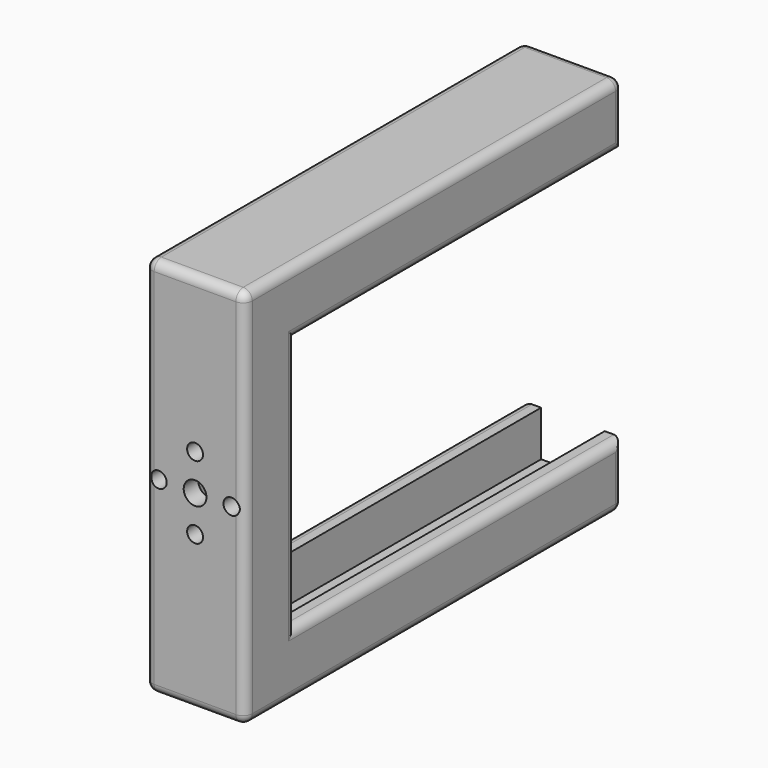
from build123d import *

# Parameters (mm, degrees)
F0_W          = 22
F0_H          = 84
F0_W_2        = 14
F0_H_2        = 76
F1_DEPTH      = 100
F2_W          = 22
F2_H          = 84
F3_DEPTH      = 4
F4_R          = 2.5
F4_R_2        = 1.75
F5_DEPTH      = 13
F6_W          = 90
F6_H          = 56
F7_DEPTH      = 22.001
F8_T1_DEPTH   = 100
F8_T3_DEPTH   = 17
F8_T5_DEPTH   = 95
F8_T7_DEPTH   = 56
F8_T9_DEPTH   = 17
F8_T11_DEPTH  = 80
F8_T13_DEPTH  = 18
F8_S17_W      = 2
F8_S17_H      = 2
F8_T18_DEPTH  = 2
F8_S23_W      = 2
F8_S23_H      = 2
F8_T24_DEPTH  = 2
F8_S29_W      = 2
F8_S29_H      = 2
F8_T30_DEPTH  = 2
F8_S35_W      = 2
F8_S35_H      = 2
F8_T36_DEPTH  = 2
F8_S41_W      = 2
F8_S41_H      = 2
F8_T42_DEPTH  = 2
F8_S47_W      = 2
F8_S47_H      = 2
F8_T48_DEPTH  = 2
F8_S53_W      = 2
F8_S53_H      = 2
F8_T54_DEPTH  = 2
F8_S59_W      = 2
F8_S59_H      = 2
F8_T60_DEPTH  = 2
F8_T67_DEPTH  = 100
F8_T71_DEPTH  = 61
F8_T78_DEPTH  = 61
F8_T82_DEPTH  = 100
F8_T89_DEPTH  = 100
F8_T93_DEPTH  = 61
F8_T100_DEPTH = 61
F8_T104_DEPTH = 100


# Not quite as in the source:
# - a fillet or chamfer that OpenCascade refuses, or shapes differently, is made with other operations: its cross-section is extruded or revolved along the edge and cut away or added


with BuildPart() as f1:
    # F0 (on Front) → F1 (new body)
    with BuildSketch(Plane.XZ):
        Rectangle(F0_W, F0_H)
        Rectangle(F0_W_2, F0_H_2, mode=Mode.SUBTRACT)
    extrude(amount=F1_DEPTH)

    # F2 (on face) → F3 (join)
    with BuildSketch(Plane.XZ.offset(100)):
        Rectangle(F2_W, F2_H)
    extrude(amount=F3_DEPTH)

    # F4 (on face) → F5 (cut)
    with BuildSketch(Plane.XZ.offset(104)):
        Circle(F4_R)
        with Locations((0, 8)):
            Circle(F4_R_2)
        with Locations((-8, 0)):
            Circle(F4_R_2)
        with Locations((0, -8)):
            Circle(F4_R_2)
        with Locations((8, 0)):
            Circle(F4_R_2)
    extrude(amount=-F5_DEPTH, mode=Mode.SUBTRACT)

    # F6 (on face) → F7 (cut, through all)
    with BuildSketch(Plane.YZ.offset(11)):
        with Locations((-45, 0)):
            Rectangle(F6_W, F6_H)
    extrude(amount=-F7_DEPTH, mode=Mode.SUBTRACT)

    # F8: fillet of radius 2 on 20 edges, made by hand

    # F8_s2 → F8_t1 (cut)
    with BuildSketch(Plane.XZ.offset(2)):
        with BuildLine():
            ThreePointArc((11, -40), (10.4142135624, -41.4142135624), (9, -42))
            Line((9, -42), (11, -42))
            Line((11, -42), (11, -40))
        make_face()
        with BuildLine():
            ThreePointArc((9, 42), (10.4142135624, 41.4142135624), (11, 40))
            Line((11, 40), (11, 42))
            Line((11, 42), (9, 42))
        make_face()
        with BuildLine():
            ThreePointArc((-11, -40), (-10.4142135624, -41.4142135624), (-9, -42))
            Line((-9, -42), (-11, -42))
            Line((-11, -42), (-11, -40))
        make_face()
        with BuildLine():
            ThreePointArc((-9, 42), (-10.4142135624, 41.4142135624), (-11, 40))
            Line((-11, 40), (-11, 42))
            Line((-11, 42), (-9, 42))
        make_face()
    extrude(amount=F8_T1_DEPTH, mode=Mode.SUBTRACT)

    # F8_s4 → F8_t3 (cut)
    with BuildSketch(Plane.XY.offset(-40)):
        with BuildLine():
            ThreePointArc((11, -2), (10.4142135624, -0.5857864376), (9, 0))
            Line((9, 0), (11, 0))
            Line((11, 0), (11, -2))
        make_face()
        with BuildLine():
            ThreePointArc((-11, -2), (-10.4142135624, -0.5857864376), (-9, 0))
            Line((-9, 0), (-11, 0))
            Line((-11, 0), (-11, -2))
        make_face()
    extrude(amount=F8_T3_DEPTH, mode=Mode.SUBTRACT)

    # F8_s6 → F8_t5 (cut)
    with BuildSketch(Plane.XZ.offset(-5)):
        with BuildLine():
            ThreePointArc((11, -30), (10.4142135624, -28.5857864376), (9, -28))
            Line((9, -28), (11, -28))
            Line((11, -28), (11, -30))
        make_face()
        with BuildLine():
            ThreePointArc((11, 30), (10.4142135624, 28.5857864376), (9, 28))
            Line((9, 28), (11, 28))
            Line((11, 28), (11, 30))
        make_face()
        with BuildLine():
            ThreePointArc((-11, 30), (-10.4142135624, 28.5857864376), (-9, 28))
            Line((-9, 28), (-11, 28))
            Line((-11, 28), (-11, 30))
        make_face()
        with BuildLine():
            ThreePointArc((-11, -30), (-10.4142135624, -28.5857864376), (-9, -28))
            Line((-9, -28), (-11, -28))
            Line((-11, -28), (-11, -30))
        make_face()
    extrude(amount=F8_T5_DEPTH, mode=Mode.SUBTRACT)

    # F8_s8 → F8_t7 (cut)
    with BuildSketch(Plane.XY.offset(-28)):
        with BuildLine():
            ThreePointArc((11, -92), (10.4142135624, -90.5857864376), (9, -90))
            Line((9, -90), (11, -90))
            Line((11, -90), (11, -92))
        make_face()
        with BuildLine():
            ThreePointArc((-11, -92), (-10.4142135624, -90.5857864376), (-9, -90))
            Line((-9, -90), (-11, -90))
            Line((-11, -90), (-11, -92))
        make_face()
    extrude(amount=F8_T7_DEPTH, mode=Mode.SUBTRACT)

    # F8_s10 → F8_t9 (cut)
    with BuildSketch(Plane.XY.offset(23)):
        with BuildLine():
            ThreePointArc((11, -2), (10.4142135624, -0.5857864376), (9, 0))
            Line((9, 0), (11, 0))
            Line((11, 0), (11, -2))
        make_face()
        with BuildLine():
            ThreePointArc((-11, -2), (-10.4142135624, -0.5857864376), (-9, 0))
            Line((-9, 0), (-11, 0))
            Line((-11, 0), (-11, -2))
        make_face()
    extrude(amount=F8_T9_DEPTH, mode=Mode.SUBTRACT)

    # F8_s12 → F8_t11 (cut)
    with BuildSketch(Plane.XY.offset(-40)):
        with BuildLine():
            ThreePointArc((11, -102), (10.4142135624, -103.4142135624), (9, -104))
            Line((9, -104), (11, -104))
            Line((11, -104), (11, -102))
        make_face()
        with BuildLine():
            ThreePointArc((-9, -104), (-10.4142135624, -103.4142135624), (-11, -102))
            Line((-11, -102), (-11, -104))
            Line((-11, -104), (-9, -104))
        make_face()
    extrude(amount=F8_T11_DEPTH, mode=Mode.SUBTRACT)

    # F8_s14 → F8_t13 (cut)
    with BuildSketch(Plane.YZ.offset(-9)):
        with BuildLine():
            ThreePointArc((-102, 42), (-103.4142135624, 41.4142135624), (-104, 40))
            Line((-104, 40), (-104, 42))
            Line((-104, 42), (-102, 42))
        make_face()
        with BuildLine():
            ThreePointArc((-2, 42), (-0.5857864376, 41.4142135624), (0, 40))
            Line((0, 40), (0, 42))
            Line((0, 42), (-2, 42))
        make_face()
        with BuildLine():
            ThreePointArc((-104, -40), (-103.4142135624, -41.4142135624), (-102, -42))
            Line((-102, -42), (-104, -42))
            Line((-104, -42), (-104, -40))
        make_face()
        with BuildLine():
            ThreePointArc((-2, -42), (-0.5857864376, -41.4142135624), (0, -40))
            Line((0, -40), (0, -42))
            Line((0, -42), (-2, -42))
        make_face()
    extrude(amount=F8_T13_DEPTH, mode=Mode.SUBTRACT)


with BuildPart() as f8_tool16:
    # F8_s17 → F8_t18 (new body)
    with BuildSketch(Plane.YZ.offset(9)):
        with Locations((-103, -41)):
            Rectangle(F8_S17_W, F8_S17_H)
    extrude(amount=F8_T18_DEPTH)

    # F8_s19 → F8_t20 (revolve, cut)
    with BuildSketch(Plane(origin=(9, -102, -40), x_dir=(0, 0.7071067812, 0.7071067812), z_dir=(0, 0.7071067812, -0.7071067812))):
        with BuildLine():
            ThreePointArc((0, -2), (2, 0), (0, 2))
            Line((0, 2), (0, -2))
        make_face()
    revolve(axis=Axis((9, -102, -40), (1, 0, 0)), mode=Mode.SUBTRACT)


with BuildPart() as f1_1:
    add(f1.part)

    # F8_t15: cut F8_tool16
    add(f8_tool16.part, mode=Mode.SUBTRACT)


with BuildPart() as f8_tool22:
    # F8_s23 → F8_t24 (new body)
    with BuildSketch(Plane.YZ.offset(9)):
        with Locations((-1, -41)):
            Rectangle(F8_S23_W, F8_S23_H)
    extrude(amount=F8_T24_DEPTH)

    # F8_s25 → F8_t26 (revolve, cut)
    with BuildSketch(Plane(origin=(9, -2, -40), x_dir=(0, -0.7071067812, 0.7071067812), z_dir=(0, 0.7071067812, 0.7071067812))):
        with BuildLine():
            ThreePointArc((0, -2), (2, 0), (0, 2))
            Line((0, 2), (0, -2))
        make_face()
    revolve(axis=Axis((9, -2, -40), (1, 0, 0)), mode=Mode.SUBTRACT)


with BuildPart() as f1_2:
    add(f1_1.part)

    # F8_t21: cut F8_tool22
    add(f8_tool22.part, mode=Mode.SUBTRACT)


with BuildPart() as f8_tool28:
    # F8_s29 → F8_t30 (new body)
    with BuildSketch(Plane.XY.offset(40)):
        with Locations((10, -1)):
            Rectangle(F8_S29_W, F8_S29_H)
    extrude(amount=F8_T30_DEPTH)

    # F8_s31 → F8_t32 (revolve, cut)
    with BuildSketch(Plane(origin=(9, -2, 40), x_dir=(-0.7071067812, -0.7071067812, 0), z_dir=(-0.7071067812, 0.7071067812, 0))):
        with BuildLine():
            ThreePointArc((0, -2), (2, 0), (0, 2))
            Line((0, 2), (0, -2))
        make_face()
    revolve(axis=Axis((9, -2, 40), (0, 0, 1)), mode=Mode.SUBTRACT)


with BuildPart() as f1_3:
    add(f1_2.part)

    # F8_t27: cut F8_tool28
    add(f8_tool28.part, mode=Mode.SUBTRACT)


with BuildPart() as f8_tool34:
    # F8_s35 → F8_t36 (new body)
    with BuildSketch(Plane.XY.offset(40)):
        with Locations((10, -103)):
            Rectangle(F8_S35_W, F8_S35_H)
    extrude(amount=F8_T36_DEPTH)

    # F8_s37 → F8_t38 (revolve, cut)
    with BuildSketch(Plane(origin=(9, -102, 40), x_dir=(-0.7071067812, 0.7071067812, 0), z_dir=(0.7071067812, 0.7071067812, 0))):
        with BuildLine():
            ThreePointArc((0, -2), (2, 0), (0, 2))
            Line((0, 2), (0, -2))
        make_face()
    revolve(axis=Axis((9, -102, 40), (0, 0, 1)), mode=Mode.SUBTRACT)


with BuildPart() as f1_4:
    add(f1_3.part)

    # F8_t33: cut F8_tool34
    add(f8_tool34.part, mode=Mode.SUBTRACT)


with BuildPart() as f8_tool40:
    # F8_s41 → F8_t42 (new body)
    with BuildSketch(Plane.XY.offset(40)):
        with Locations((-10, -1)):
            Rectangle(F8_S41_W, F8_S41_H)
    extrude(amount=F8_T42_DEPTH)

    # F8_s43 → F8_t44 (revolve, cut)
    with BuildSketch(Plane(origin=(-9, -2, 40), x_dir=(0.7071067812, -0.7071067812, 0), z_dir=(-0.7071067812, -0.7071067812, 0))):
        with BuildLine():
            ThreePointArc((0, -2), (2, 0), (0, 2))
            Line((0, 2), (0, -2))
        make_face()
    revolve(axis=Axis((-9, -2, 40), (0, 0, 1)), mode=Mode.SUBTRACT)


with BuildPart() as f1_5:
    add(f1_4.part)

    # F8_t39: cut F8_tool40
    add(f8_tool40.part, mode=Mode.SUBTRACT)


with BuildPart() as f8_tool46:
    # F8_s47 → F8_t48 (new body)
    with BuildSketch(Plane.YZ.offset(-9)):
        with Locations((-1, -41)):
            Rectangle(F8_S47_W, F8_S47_H)
    extrude(amount=-F8_T48_DEPTH)

    # F8_s49 → F8_t50 (revolve, cut)
    with BuildSketch(Plane(origin=(-9, -2, -40), x_dir=(0, -0.7071067812, 0.7071067812), z_dir=(0, -0.7071067812, -0.7071067812))):
        with BuildLine():
            ThreePointArc((0, -2), (2, 0), (0, 2))
            Line((0, 2), (0, -2))
        make_face()
    revolve(axis=Axis((-9, -2, -40), (-1, 0, 0)), mode=Mode.SUBTRACT)


with BuildPart() as f1_6:
    add(f1_5.part)

    # F8_t45: cut F8_tool46
    add(f8_tool46.part, mode=Mode.SUBTRACT)


with BuildPart() as f8_tool52:
    # F8_s53 → F8_t54 (new body)
    with BuildSketch(Plane.XZ.offset(102)):
        with Locations((-10, -41)):
            Rectangle(F8_S53_W, F8_S53_H)
    extrude(amount=F8_T54_DEPTH)

    # F8_s55 → F8_t56 (revolve, cut)
    with BuildSketch(Plane(origin=(-9, -102, -40), x_dir=(0.7071067812, 0, 0.7071067812), z_dir=(0.7071067812, 0, -0.7071067812))):
        with BuildLine():
            ThreePointArc((0, -2), (2, 0), (0, 2))
            Line((0, 2), (0, -2))
        make_face()
    revolve(axis=Axis((-9, -102, -40), (0, -1, 0)), mode=Mode.SUBTRACT)


with BuildPart() as f1_7:
    add(f1_6.part)

    # F8_t51: cut F8_tool52
    add(f8_tool52.part, mode=Mode.SUBTRACT)


with BuildPart() as f8_tool58:
    # F8_s59 → F8_t60 (new body)
    with BuildSketch(Plane.XY.offset(40)):
        with Locations((-10, -103)):
            Rectangle(F8_S59_W, F8_S59_H)
    extrude(amount=F8_T60_DEPTH)

    # F8_s61 → F8_t62 (revolve, cut)
    with BuildSketch(Plane(origin=(-9, -102, 40), x_dir=(0.7071067812, 0.7071067812, 0), z_dir=(0.7071067812, -0.7071067812, 0))):
        with BuildLine():
            ThreePointArc((0, -2), (2, 0), (0, 2))
            Line((0, 2), (0, -2))
        make_face()
    revolve(axis=Axis((-9, -102, 40), (0, 0, 1)), mode=Mode.SUBTRACT)


with BuildPart() as f1_8:
    add(f1_7.part)

    # F8_t57: cut F8_tool58
    add(f8_tool58.part, mode=Mode.SUBTRACT)


with BuildPart() as f8_tool65:
    # F8_s66 → F8_t67 (new body)
    with BuildSketch(Plane.XZ.offset(95)):
        with BuildLine():
            ThreePointArc((11, -30), (10.4142135624, -28.5857864376), (9, -28))
            Line((9, -28), (11, -28))
            Line((11, -28), (11, -30))
        make_face()
    extrude(amount=-F8_T67_DEPTH)

    split(bisect_by=Plane.XZ.offset(90), keep=Keep.TOP)


with BuildPart() as f8_tool69:
    # F8_s70 → F8_t71 (new body)
    with BuildSketch(Plane.XY.offset(28)):
        with BuildLine():
            ThreePointArc((11, -92), (10.4142135624, -90.5857864376), (9, -90))
            Line((9, -90), (11, -90))
            Line((11, -90), (11, -92))
        make_face()
    extrude(amount=-F8_T71_DEPTH)

    split(bisect_by=Plane.XY.offset(-28), keep=Keep.BOTTOM)


with BuildPart() as f8_tool65_1:
    add(f8_tool65.part)

    # F8_t73: intersect F8_tool69
    add(f8_tool69.part, mode=Mode.INTERSECT)


with BuildPart() as f1_9:
    add(f1_8.part)

    # F8_t63: cut F8_tool65
    add(f8_tool65_1.part, mode=Mode.SUBTRACT)


with BuildPart() as f8_tool76:
    # F8_s77 → F8_t78 (new body)
    with BuildSketch(Plane.XY.offset(33)):
        with BuildLine():
            ThreePointArc((11, -92), (10.4142135624, -90.5857864376), (9, -90))
            Line((9, -90), (11, -90))
            Line((11, -90), (11, -92))
        make_face()
    extrude(amount=-F8_T78_DEPTH)

    split(bisect_by=Plane.XY.offset(28), keep=Keep.TOP)


with BuildPart() as f8_tool80:
    # F8_s81 → F8_t82 (new body)
    with BuildSketch(Plane.XZ.offset(-5)):
        with BuildLine():
            ThreePointArc((11, 30), (10.4142135624, 28.5857864376), (9, 28))
            Line((9, 28), (11, 28))
            Line((11, 28), (11, 30))
        make_face()
    extrude(amount=F8_T82_DEPTH)

    split(bisect_by=Plane.XZ.offset(90), keep=Keep.TOP)


with BuildPart() as f8_tool76_1:
    add(f8_tool76.part)

    # F8_t84: intersect F8_tool80
    add(f8_tool80.part, mode=Mode.INTERSECT)


with BuildPart() as f1_10:
    add(f1_9.part)

    # F8_t74: cut F8_tool76
    add(f8_tool76_1.part, mode=Mode.SUBTRACT)


with BuildPart() as f8_tool87:
    # F8_s88 → F8_t89 (new body)
    with BuildSketch(Plane.XZ.offset(-5)):
        with BuildLine():
            ThreePointArc((-11, 30), (-10.4142135624, 28.5857864376), (-9, 28))
            Line((-9, 28), (-11, 28))
            Line((-11, 28), (-11, 30))
        make_face()
    extrude(amount=F8_T89_DEPTH)

    split(bisect_by=Plane.XZ.offset(90), keep=Keep.TOP)


with BuildPart() as f8_tool91:
    # F8_s92 → F8_t93 (new body)
    with BuildSketch(Plane.XY.offset(33)):
        with BuildLine():
            ThreePointArc((-11, -92), (-10.4142135624, -90.5857864376), (-9, -90))
            Line((-9, -90), (-11, -90))
            Line((-11, -90), (-11, -92))
        make_face()
    extrude(amount=-F8_T93_DEPTH)

    split(bisect_by=Plane.XY.offset(28), keep=Keep.TOP)


with BuildPart() as f8_tool87_1:
    add(f8_tool87.part)

    # F8_t95: intersect F8_tool91
    add(f8_tool91.part, mode=Mode.INTERSECT)


with BuildPart() as f1_11:
    add(f1_10.part)

    # F8_t85: cut F8_tool87
    add(f8_tool87_1.part, mode=Mode.SUBTRACT)


with BuildPart() as f8_tool98:
    # F8_s99 → F8_t100 (new body)
    with BuildSketch(Plane.XY.offset(28)):
        with BuildLine():
            ThreePointArc((-11, -92), (-10.4142135624, -90.5857864376), (-9, -90))
            Line((-9, -90), (-11, -90))
            Line((-11, -90), (-11, -92))
        make_face()
    extrude(amount=-F8_T100_DEPTH)

    split(bisect_by=Plane.XY.offset(-28), keep=Keep.BOTTOM)


with BuildPart() as f8_tool102:
    # F8_s103 → F8_t104 (new body)
    with BuildSketch(Plane.XZ.offset(95)):
        with BuildLine():
            ThreePointArc((-11, -30), (-10.4142135624, -28.5857864376), (-9, -28))
            Line((-9, -28), (-11, -28))
            Line((-11, -28), (-11, -30))
        make_face()
    extrude(amount=-F8_T104_DEPTH)

    split(bisect_by=Plane.XZ.offset(90), keep=Keep.TOP)


with BuildPart() as f8_tool98_1:
    add(f8_tool98.part)

    # F8_t106: intersect F8_tool102
    add(f8_tool102.part, mode=Mode.INTERSECT)


with BuildPart() as f1_12:
    add(f1_11.part)

    # F8_t96: cut F8_tool98
    add(f8_tool98_1.part, mode=Mode.SUBTRACT)


solid = f1_12.part
